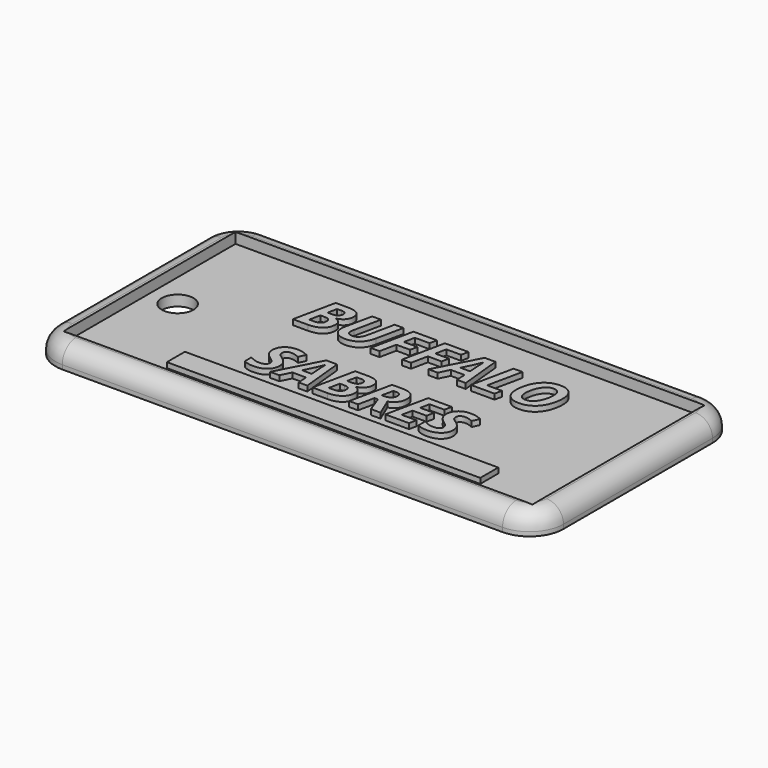
from build123d import *

# Parameters (mm, degrees)
F0_W         = 70.358
F0_H         = 32.258
F0_R         = 2.38125
F1_DEPTH     = 1.5875
F0_W_2       = 76.2
F0_H_2       = 38.1
F2_DEPTH     = 3.175
F3_R         = 5.08
F4_T1_DEPTH  = 66.04
F4_T3_DEPTH  = 27.94
F4_T6_ANGLE  = 90
F4_T8_ANGLE  = 90
F4_T10_ANGLE = 90
F4_T12_ANGLE = 90
F5_W         = 47.0107197762
F5_H         = 3.3744266257
F5_TEXT_SIZE = 8.8960233491
F6_DEPTH     = 0.79375


# Not quite as in the source:
# - a fillet or chamfer that OpenCascade refuses, or shapes differently, is made with other operations: its cross-section is extruded or revolved along the edge and cut away or added
# - Text() gives the source's letters only with a copy of the font that has no kerning and outlines rounded to 1/6400 em; it was checked with that copy


with BuildPart() as f1:
    # F0 (on Top) → F1 (new body)
    with BuildSketch(Plane.XY):
        with Locations((38.1, 19.05)):
            Rectangle(F0_W, F0_H)
        with Locations((7.14375, 19.05)):
            Circle(F0_R, mode=Mode.SUBTRACT)
    extrude(amount=F1_DEPTH)

    # F0 (on Top) → F2 (join)
    with BuildSketch(Plane.XY):
        with Locations((38.1, 19.05)):
            Rectangle(F0_W_2, F0_H_2)
        with Locations((38.1, 19.05)):
            Rectangle(F0_W, F0_H, mode=Mode.SUBTRACT)
    extrude(amount=F2_DEPTH)

    # F3
    f3_edges = [f1.edges().sort_by_distance(p)[0] for p in [
        (76.2, 0, 1.5875),
        (0, 0, 1.5875),
        (76.2, 38.1, 1.5875),
        (0, 38.1, 1.5875),
    ]]
    fillet(f3_edges, radius=F3_R)

    # F4: fillet of radius 2.54 on 8 edges, made by hand

    # F4_s2 → F4_t1 (cut)
    with BuildSketch(Plane.YZ.offset(5.08)):
        with BuildLine():
            ThreePointArc((0, 0.635), (0.7439487758, 2.4310512242), (2.54, 3.175))
            Line((2.54, 3.175), (0, 3.175))
            Line((0, 3.175), (0, 0.635))
        make_face()
        with BuildLine():
            ThreePointArc((38.1, 0.635), (37.3560512242, 2.4310512242), (35.56, 3.175))
            Line((35.56, 3.175), (38.1, 3.175))
            Line((38.1, 3.175), (38.1, 0.635))
        make_face()
    extrude(amount=F4_T1_DEPTH, mode=Mode.SUBTRACT)

    # F4_s4 → F4_t3 (cut)
    with BuildSketch(Plane.XZ.offset(-33.02)):
        with BuildLine():
            ThreePointArc((0, 0.635), (0.7439487758, 2.4310512242), (2.54, 3.175))
            Line((2.54, 3.175), (0, 3.175))
            Line((0, 3.175), (0, 0.635))
        make_face()
        with BuildLine():
            ThreePointArc((76.2, 0.635), (75.4560512242, 2.4310512242), (73.66, 3.175))
            Line((73.66, 3.175), (76.2, 3.175))
            Line((76.2, 3.175), (76.2, 0.635))
        make_face()
    extrude(amount=F4_T3_DEPTH, mode=Mode.SUBTRACT)

    # F4_s5 → F4_t6 (revolve, cut)
    with BuildSketch(Plane.XZ.offset(-33.02)):
        with BuildLine():
            ThreePointArc((0, 0.635), (0.7439487758, 2.4310512242), (2.54, 3.175))
            Line((2.54, 3.175), (0, 3.175))
            Line((0, 3.175), (0, 0.635))
        make_face()
    revolve(axis=Axis((5.08, 33.02, 3.175), (0, 0, -1)), revolution_arc=F4_T6_ANGLE, mode=Mode.SUBTRACT)

    # F4_s7 → F4_t8 (revolve, cut)
    with BuildSketch(Plane.XZ.offset(-5.08)):
        with BuildLine():
            ThreePointArc((0, 0.635), (0.7439487758, 2.4310512242), (2.54, 3.175))
            Line((2.54, 3.175), (0, 3.175))
            Line((0, 3.175), (0, 0.635))
        make_face()
    revolve(axis=Axis((5.08, 5.08, 3.175), (0, 0, 1)), revolution_arc=F4_T8_ANGLE, mode=Mode.SUBTRACT)

    # F4_s9 → F4_t10 (revolve, cut)
    with BuildSketch(Plane.XZ.offset(-33.02)):
        with BuildLine():
            ThreePointArc((76.2, 0.635), (75.4560512242, 2.4310512242), (73.66, 3.175))
            Line((73.66, 3.175), (76.2, 3.175))
            Line((76.2, 3.175), (76.2, 0.635))
        make_face()
    revolve(axis=Axis((71.12, 33.02, 3.175), (0, 0, 1)), revolution_arc=F4_T10_ANGLE, mode=Mode.SUBTRACT)

    # F4_s11 → F4_t12 (revolve, cut)
    with BuildSketch(Plane.YZ.offset(71.12)):
        with BuildLine():
            ThreePointArc((0, 0.635), (0.7439487758, 2.4310512242), (2.54, 3.175))
            Line((2.54, 3.175), (0, 3.175))
            Line((0, 3.175), (0, 0.635))
        make_face()
    revolve(axis=Axis((71.12, 5.08, 3.175), (0, 0, 1)), revolution_arc=F4_T12_ANGLE, mode=Mode.SUBTRACT)

    # F5 (on face) → F6 (join)
    with BuildSketch(Plane.XY.offset(1.5875)):
        with Locations((39.8425683379, 7.2289011441)):
            Rectangle(F5_W, F5_H)
        with Locations((20.8230056472, 23.2708923315)):
            Text('BUFFALO', F5_TEXT_SIZE, font='Open Sans', font_style=FontStyle.BOLDITALIC, text_align=(TextAlign.LEFT, TextAlign.BOTTOM))
        with Locations((23.1345817143, 11.1723005767)):
            Text('SABRES', F5_TEXT_SIZE, font='Open Sans', font_style=FontStyle.BOLDITALIC, text_align=(TextAlign.LEFT, TextAlign.BOTTOM))
    extrude(amount=F6_DEPTH)


solid = f1.part
